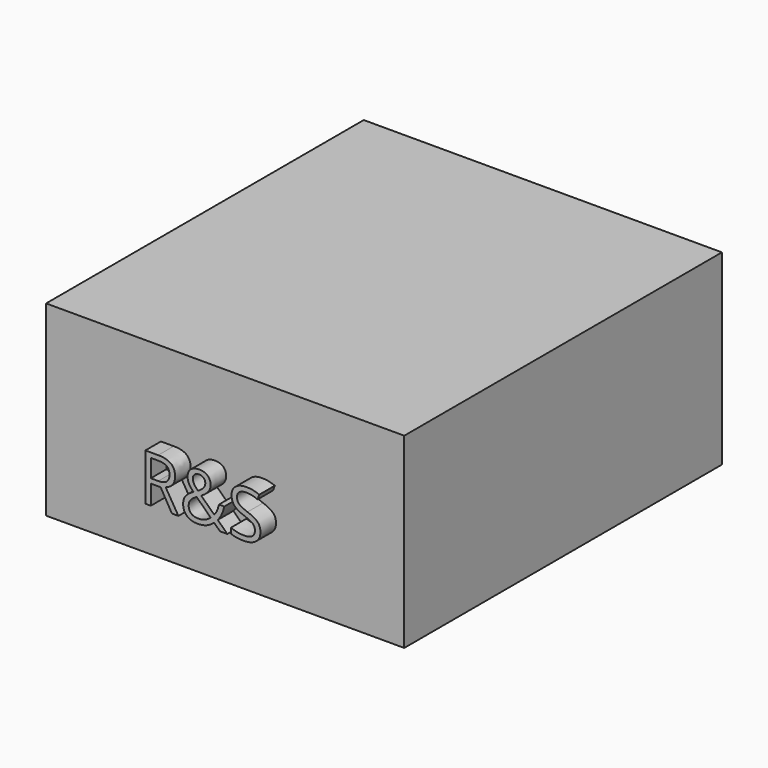
from build123d import *

# Parameters (mm, degrees)
F0_W         = 460
F0_H         = 240
F1_DEPTH     = 255
F2_TEXT_SIZE = 84.4085537311
F3_DEPTH     = 25


# Not quite as in the source:
# - Text() gives the source's letters only with a copy of the font that has no kerning and outlines rounded to 1/6400 em; it was checked with that copy


with BuildPart() as f1:
    # F0 (on Front) → F1 (new body, symmetric)
    with BuildSketch(Plane.XZ):
        Rectangle(F0_W, F0_H)
    extrude(amount=F1_DEPTH, both=True)

    # F2 (on face) → F3 (join)
    with BuildSketch(Plane.XZ.offset(255)):
        with Locations((-90.7921791077, -48.3831651509)):
            Text('R&S', F2_TEXT_SIZE, font='Open Sans', text_align=(TextAlign.LEFT, TextAlign.BOTTOM))
    extrude(amount=F3_DEPTH)


solid = f1.part
